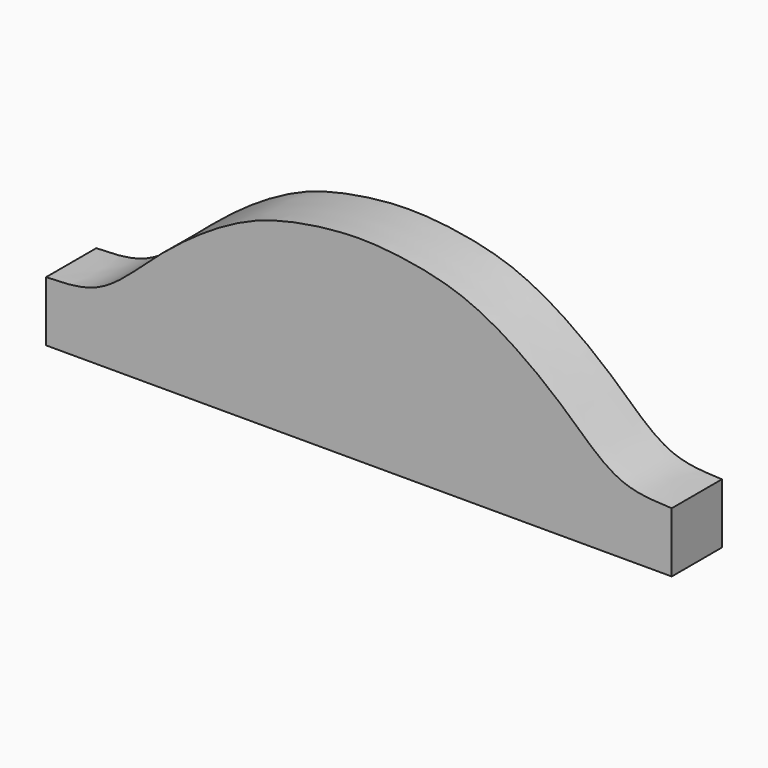
from build123d import *

# Parameters (mm, degrees)
F2_DEPTH = 2.2


# Not quite as in the source:
# - the dataset's text gives a spline's control points without its knots; the knots are read off the source's solid


with BuildPart() as f2:
    # F1 (on Front) → F2 (new body)
    with BuildSketch(Plane.XZ):
        with BuildLine():
            add(Edge.make_bspline(
                [(-11, -1.3276004465), (-10.3729307876, -1.3132402784), (-9.0451139721, -1.2828327097), (-7.3416600471, 0.4414314678), (-5.5526562986, 1.8457039738), (-3.7123096789, 2.8814024285), (-1.8449980561, 3.3196881712), (-0.0113724229, 3.5001251182), (1.8347031854, 3.3201000435), (3.7002930815, 2.8815464529), (5.5422002335, 1.8450988588), (7.3286228258, 0.443839629), (9.0337178792, -1.2845021367), (10.3334013638, -1.2967170507), (10.9408724309, -1.3276004465)],
                knots=[0, 0, 0, 0, 0.0794256135, 0.1682210626, 0.2571509511, 0.3412658537, 0.421535998, 0.500390533, 0.5794847456, 0.6597547285, 0.7438697718, 0.83279966, 0.9215951091, 1, 1, 1, 1], degree=3))
            Line((-11, -1.3276004465), (-11, -3.4346309038))
            Line((-11, -3.4346309038), (10.9408724309, -3.4346309038))
            Line((10.9408724309, -3.4346309038), (10.9408724309, -1.3276004465))
        make_face()
    extrude(amount=F2_DEPTH)


solid = f2.part
